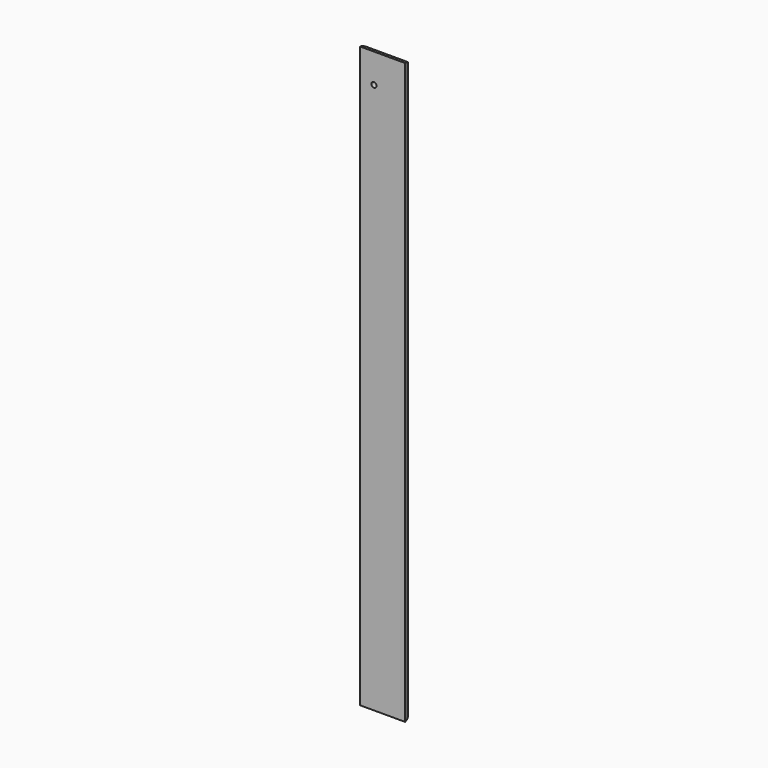
from build123d import *

# Parameters (mm, degrees)
F0_W        = 88.9
F0_H        = 1140
F0_R        = 5
F1_DEPTH    = 38.1
F2_T1_DEPTH = 1382.8162885805
F2_T3_DEPTH = 331.7162885805


# Not quite as in the source:
# - a fillet or chamfer that OpenCascade refuses, or shapes differently, is made with other operations: its cross-section is extruded or revolved along the edge and cut away or added


with BuildPart() as f1:
    # F0 (on Front) → F1 (new body)
    with BuildSketch(Plane.XZ):
        with Locations((-1911.2522443051, 3.6825537682)):
            Rectangle(F0_W, F0_H)
        with Locations((-1928.2022443051, 516.0674452782)):
            Circle(F0_R, mode=Mode.SUBTRACT)
    extrude(amount=F1_DEPTH)

    # F2: fillet of radius 50 on 2 edges, made by hand

    # F2_s2 → F2_t1 (cut)
    with BuildSketch(Plane.XY.offset(-687.7255905221)):
        with BuildLine():
            ThreePointArc((-1866.8022443051, -38.1), (-1884.5029032971, -10.6617234745), (-1915.3655020212, 0))
            Line((-1915.3655020212, 0), (-1866.8022443051, 0))
            Line((-1866.8022443051, 0), (-1866.8022443051, -38.1))
        make_face()
    extrude(amount=F2_T1_DEPTH, mode=Mode.SUBTRACT)

    # F2_s4 → F2_t3 (cut)
    with BuildSketch(Plane.YZ.offset(-2077.1103885953)):
        with BuildLine():
            ThreePointArc((-38.1, 573.6825537682), (-10.6617234745, 555.9818947761), (0, 525.1192960521))
            Line((0, 525.1192960521), (0, 573.6825537682))
            Line((0, 573.6825537682), (-38.1, 573.6825537682))
        make_face()
    extrude(amount=F2_T3_DEPTH, mode=Mode.SUBTRACT)


solid = f1.part
